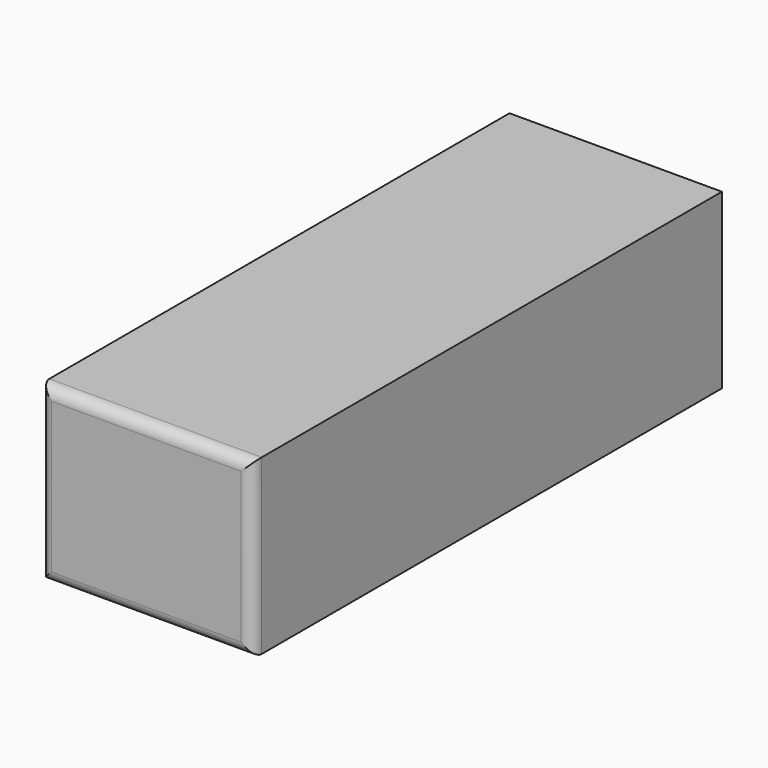
from build123d import *

# Parameters (mm, degrees)
F0_W      = 37.3
F0_H      = 30.4
F0_W_2    = 32.3
F0_H_2    = 25.4
F1_DEPTH  = 100
F2_W      = 37.3
F2_H      = 30.4
F3_DEPTH  = 3
F4_R      = 2
F5_R      = 1.75
F6_R      = 1.75
F7_DEPTH  = 1
F8_R      = 0.99999
F9_R      = 1.75
F10_DEPTH = 1
F11_R     = 0.99999
F12_W     = 32.3
F12_H     = 2
F13_DEPTH = 1
F14_W     = 32.3
F14_H     = 2
F15_DEPTH = 1


# Not quite as in the source:
# - a fillet or chamfer is up to 0.001 mm smaller than in the source, because OpenCascade refuses the exact size


with BuildPart() as f1:
    # F0 (on Front) → F1 (new body)
    with BuildSketch(Plane.XZ):
        with Locations((-0.3367068468, 2.3746712297)):
            Rectangle(F0_W, F0_H)
        with Locations((-0.3367068468, 2.3746712297)):
            Rectangle(F0_W_2, F0_H_2, mode=Mode.SUBTRACT)
    extrude(amount=F1_DEPTH)

    # F2 (on face) → F3 (join)
    with BuildSketch(Plane.XZ.offset(100)):
        with Locations((-0.3367068468, 2.3746712297)):
            Rectangle(F2_W, F2_H)
    extrude(amount=F3_DEPTH)

    # F4
    f4_edges = [f1.edges().sort_by_distance(p)[0] for p in [
        (-0.336707, -103, 17.574671),
        (-18.986707, -103, 2.374671),
        (-0.336707, -103, -12.825329),
        (18.313293, -103, 2.374671),
    ]]
    fillet(f4_edges, radius=F4_R)

    # F5
    f5_edges = [f1.edges().sort_by_distance(p)[0] for p in [
        (15.813293, 0, 2.374671),
        (-0.336707, 0, 15.074671),
        (-16.486707, 0, 2.374671),
        (-0.336707, 0, -10.325329),
    ]]
    fillet(f5_edges, radius=F5_R)

    # F6 (on face) → F7 (cut)
    with BuildSketch(Plane.XY.offset(-10.3253287703)):
        with Locations((-0.3367068468, -17.5)):
            Circle(F6_R)
    extrude(amount=-F7_DEPTH, mode=Mode.SUBTRACT)

    # F8 (radius 1 in the source; OpenCascade refuses exactly that, so slightly less here)
    f8_edges = [f1.edges().sort_by_distance(p)[0] for p in [
        (-2.086707, -17.5, -11.325329),
    ]]
    fillet(f8_edges, radius=F8_R)

    # F9 (on face) → F10 (cut)
    with BuildSketch(Plane(origin=(0, 0, 15.0746712297), x_dir=(1, 0, 0), z_dir=(0, 0, -1))):
        with Locations((-0.3367068468, 17.5)):
            Circle(F9_R)
    extrude(amount=-F10_DEPTH, mode=Mode.SUBTRACT)

    # F11 (radius 1 in the source; OpenCascade refuses exactly that, so slightly less here)
    f11_edges = [f1.edges().sort_by_distance(p)[0] for p in [
        (-2.086707, -17.5, 16.074671),
    ]]
    fillet(f11_edges, radius=F11_R)

    # F12 (on face) → F13 (join)
    with BuildSketch(Plane.XY.offset(-10.3253287703)):
        with Locations((-0.3367068468, -45.3)):
            Rectangle(F12_W, F12_H)
    extrude(amount=F13_DEPTH)

    # F14 (on face) → F15 (join)
    with BuildSketch(Plane(origin=(0, 0, 15.0746712297), x_dir=(1, 0, 0), z_dir=(0, 0, -1))):
        with Locations((-0.3367068468, 45.3)):
            Rectangle(F14_W, F14_H)
    extrude(amount=F15_DEPTH)


solid = f1.part
